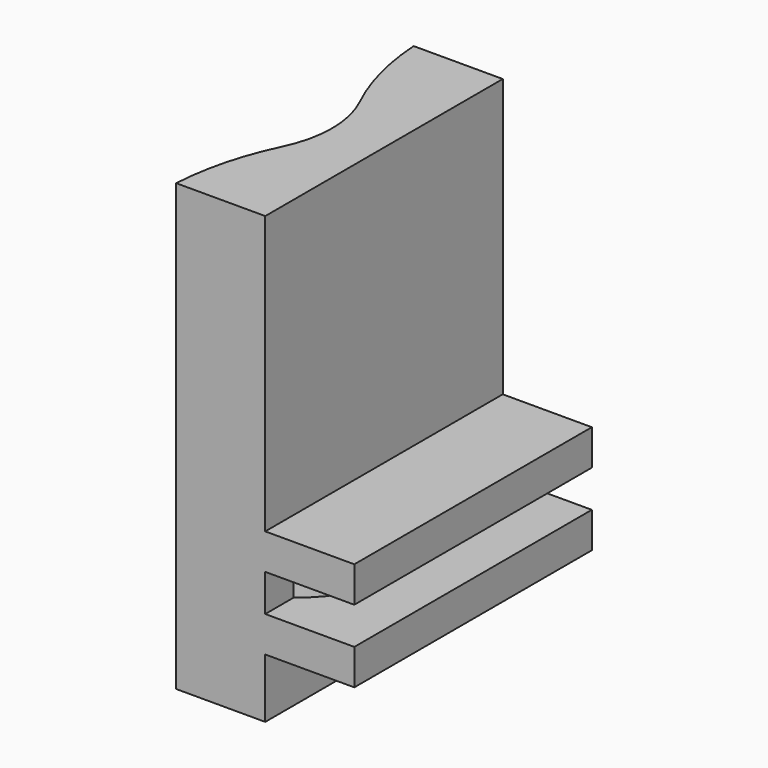
from build123d import *

# Parameters (mm, degrees)
F1_DEPTH    = 25.4
F2_T1_DEPTH = 53.4024208572
F3_DEPTH    = 10.16
F4_DEPTH    = 2.54
F5_W        = 25.4
F5_H        = 3.048
F6_DEPTH    = 7.62
F8_DEPTH    = 5.08


# Not quite as in the source:
# - a fillet or chamfer that OpenCascade refuses, or shapes differently, is made with other operations: its cross-section is extruded or revolved along the edge and cut away or added


with BuildPart() as f1:
    # F0 (on Top) → F1 (new body)
    with BuildSketch(Plane.XY):
        with BuildLine():
            Line((-3.81, -12.7), (3.81, -12.7))
            Line((3.81, -12.7), (3.81, 12.7))
            Line((3.81, 12.7), (-3.81, 12.7))
            Line((-3.81, 12.7), (-3.81, 7.0995158286))
            ThreePointArc((-3.81, 7.0995158286), (-1.4649043996, 3.8885649667), (-0.635, 0))
            ThreePointArc((-0.635, 0), (-1.4649043996, -3.8885649667), (-3.81, -7.0995158286))
            Line((-3.81, -7.0995158286), (-3.81, -12.7))
        make_face()
    extrude(amount=F1_DEPTH)

    # F2: fillet of radius 22.86 on 2 edges, made by hand

    # F2_s2 → F2_t1 (cut)
    with BuildSketch(Plane.XY.offset(-14.0012104286)):
        with BuildLine():
            ThreePointArc((-3.81, 12.7), (-3.1136000163, 8.3102394823), (-1.5809070588, 4.1382108824))
            ThreePointArc((-1.5809070588, 4.1382108824), (-2.5500206467, 5.7283365162), (-3.81, 7.0995158286))
            Line((-3.81, 7.0995158286), (-3.81, 12.7))
        make_face()
        with BuildLine():
            ThreePointArc((-3.81, -12.7), (-3.1136000163, -8.3102394823), (-1.5809070588, -4.1382108824))
            ThreePointArc((-1.5809070588, -4.1382108824), (-2.5500206467, -5.7283365162), (-3.81, -7.0995158286))
            Line((-3.81, -7.0995158286), (-3.81, -12.7))
        make_face()
    extrude(amount=F2_T1_DEPTH, mode=Mode.SUBTRACT)

    # F3 (add): a face of the model
    f3_faces = [f1.faces().sort_by_distance(p)[0] for p in [
        (0.6414875327, 0, 25.4),
    ]]
    extrude(f3_faces, amount=F3_DEPTH)

    # F4 (add): a face of the model
    f4_faces = [f1.faces().sort_by_distance(p)[0] for p in [
        (0.6414875327, 0, 35.56),
    ]]
    extrude(f4_faces, amount=F4_DEPTH)

    # F5 (on face) → F6 (join)
    with BuildSketch(Plane.YZ.offset(3.81)):
        with Locations((0, 12.827)):
            Rectangle(F5_W, F5_H)
        with Locations((0, 6.604)):
            Rectangle(F5_W, F5_H)
    extrude(amount=F6_DEPTH)

    # F7 (on face) → F8 (join)
    with BuildSketch(Plane.XY.offset(8.128)):
        with BuildLine():
            ThreePointArc((3.81, -9.652), (6.427457728, -6.515728864), (7.366, -2.54))
            ThreePointArc((7.366, -2.54), (6.427457728, 1.435728864), (3.81, 4.572))
            Line((3.81, 4.572), (3.81, -9.652))
        make_face()
    extrude(amount=F8_DEPTH)


solid = f1.part
